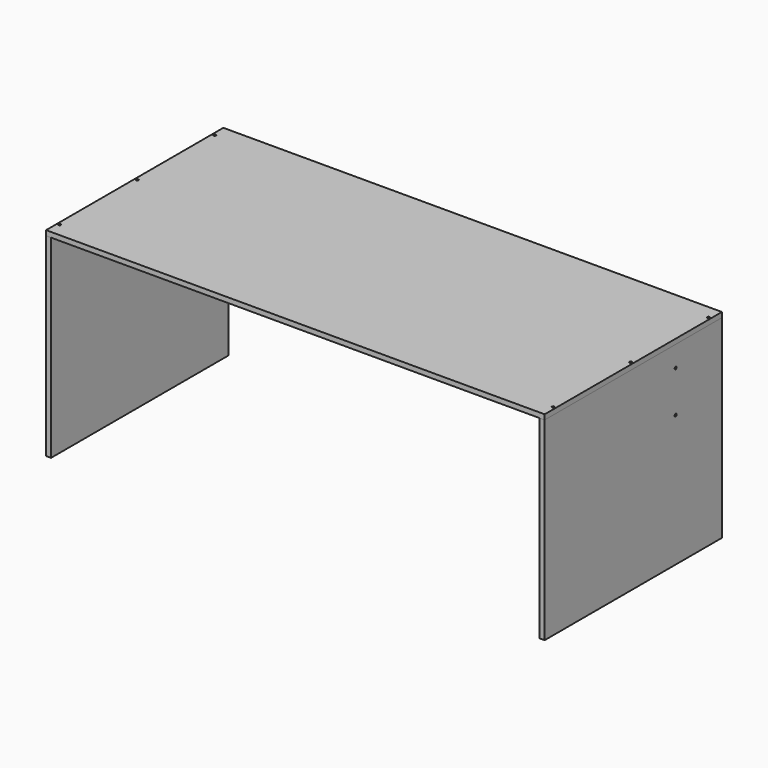
from build123d import *

# Parameters (mm, degrees)
F1_DEPTH          = 800
F0_W              = 18
F0_H              = 700
F2_DEPTH          = 800
F3_W              = 1764
F3_H              = 18
F4_DEPTH          = 300
F6_D              = 4
F6_DEPTH          = 20
F6_CSINK_D        = 8.96
F6_CSINK_ANGLE    = 90
F6_TIP            = 1.2017212381
F6_2_D            = 4
F6_2_DEPTH        = 20
F6_2_CSINK_D      = 8.96
F6_2_CSINK_ANGLE  = 90
F6_2_TIP          = 1.2017212381
F6_3_D            = 4
F6_3_DEPTH        = 20
F6_3_CSINK_D      = 8.96
F6_3_CSINK_ANGLE  = 90
F6_3_TIP          = 1.2017212381
F8_D              = 4
F8_DEPTH          = 40
F8_CSINK_D        = 8.96
F8_CSINK_ANGLE    = 90
F8_TIP            = 1.2017212381
F8_2_D            = 4
F8_2_DEPTH        = 40
F8_2_CSINK_D      = 8.96
F8_2_CSINK_ANGLE  = 90
F8_2_TIP          = 1.2017212381
F10_D             = 4
F10_DEPTH         = 40
F10_CSINK_D       = 8.96
F10_CSINK_ANGLE   = 90
F10_TIP           = 1.2017212381
F10_2_D           = 4
F10_2_DEPTH       = 40
F10_2_CSINK_D     = 8.96
F10_2_CSINK_ANGLE = 90
F10_2_TIP         = 1.2017212381
F12_D             = 3
F12_DEPTH         = 1
F12_TIP           = 0.9012909285
F12_2_D           = 3
F12_2_DEPTH       = 1
F12_2_TIP         = 0.9012909285


# Not quite as in the source:
# - a feature names something its author has since deleted; it is built from what else it names


with BuildPart() as f1:
    # F0 (on Front) → F1 (new body)
    with BuildSketch(Plane.XZ):
        Polygon((0, 18), (0, 0), (18, 0), (1782, 0), (1800, 0), (1800, 18), align=None)
    extrude(amount=-F1_DEPTH)

    # F6
    with Locations(Plane.XY.offset(18)):
        with Locations((9, 750), (9, 400), (9, 50), (1791, 750), (1791, 400), (1791, 50)):
            CounterSinkHole(F6_D / 2, F6_CSINK_D / 2, depth=F6_DEPTH, counter_sink_angle=F6_CSINK_ANGLE)
            with Locations((0, 0, -(F6_DEPTH + F6_TIP / 2))):  # 118° drill point
                Cone(0, F6_D / 2, F6_TIP, mode=Mode.SUBTRACT)


with BuildPart() as f2:
    # F0 (on Front) → F2 (new body)
    with BuildSketch(Plane.XZ):
        with Locations((9, -350)):
            Rectangle(F0_W, F0_H)
    extrude(amount=-F2_DEPTH)

    # F6#2
    with Locations(Plane.XY.offset(18)):
        with Locations((9, 750), (9, 400), (9, 50), (1791, 750), (1791, 400), (1791, 50)):
            CounterSinkHole(F6_2_D / 2, F6_2_CSINK_D / 2, depth=F6_2_DEPTH, counter_sink_angle=F6_2_CSINK_ANGLE)
            with Locations((0, 0, -(F6_2_DEPTH + F6_2_TIP / 2))):  # 118° drill point
                Cone(0, F6_2_D / 2, F6_2_TIP, mode=Mode.SUBTRACT)

    # F8
    with Locations(Plane(origin=(0, 0, 0), x_dir=(0, -1, 0), z_dir=(-1, 0, 0))):
        with Locations((-591, -75), (-591, -225)):
            CounterSinkHole(F8_D / 2, F8_CSINK_D / 2, depth=F8_DEPTH, counter_sink_angle=F8_CSINK_ANGLE)
            with Locations((0, 0, -(F8_DEPTH + F8_TIP / 2))):  # 118° drill point
                Cone(0, F8_D / 2, F8_TIP, mode=Mode.SUBTRACT)

    # F12
    with Locations(Plane(origin=(0, 0, -700), x_dir=(1, 0, 0), z_dir=(0, 0, -1))):
        with Locations((1791, -30), (1791, -770), (9, -30), (9, -770)):
            Hole(F12_D / 2, depth=F12_DEPTH)
            with Locations((0, 0, -(F12_DEPTH + F12_TIP / 2))):  # 118° drill point
                Cone(0, F12_D / 2, F12_TIP, mode=Mode.SUBTRACT)


with BuildPart() as f2b:
    # F0 (on Front) → F2, piece 2 (new body)
    with BuildSketch(Plane.XZ):
        with Locations((1791, -350)):
            Rectangle(F0_W, F0_H)
    extrude(amount=-F2_DEPTH)

    # F6#3
    with Locations(Plane.XY.offset(18)):
        with Locations((9, 750), (9, 400), (9, 50), (1791, 750), (1791, 400), (1791, 50)):
            CounterSinkHole(F6_3_D / 2, F6_3_CSINK_D / 2, depth=F6_3_DEPTH, counter_sink_angle=F6_3_CSINK_ANGLE)
            with Locations((0, 0, -(F6_3_DEPTH + F6_3_TIP / 2))):  # 118° drill point
                Cone(0, F6_3_D / 2, F6_3_TIP, mode=Mode.SUBTRACT)

    # F10
    with Locations(Plane.YZ.offset(1800)):
        with Locations((591, -75), (591, -225)):
            CounterSinkHole(F10_D / 2, F10_CSINK_D / 2, depth=F10_DEPTH, counter_sink_angle=F10_CSINK_ANGLE)
            with Locations((0, 0, -(F10_DEPTH + F10_TIP / 2))):  # 118° drill point
                Cone(0, F10_D / 2, F10_TIP, mode=Mode.SUBTRACT)

    # F12#2
    with Locations(Plane(origin=(0, 0, -700), x_dir=(1, 0, 0), z_dir=(0, 0, -1))):
        with Locations((1791, -30), (1791, -770), (9, -30), (9, -770)):
            Hole(F12_2_D / 2, depth=F12_2_DEPTH)
            with Locations((0, 0, -(F12_2_DEPTH + F12_2_TIP / 2))):  # 118° drill point
                Cone(0, F12_2_D / 2, F12_2_TIP, mode=Mode.SUBTRACT)


with BuildPart() as f4:
    # F3 (on face) → F4 (new body)
    with BuildSketch(Plane(origin=(0, 0, 0), x_dir=(1, 0, 0), z_dir=(0, 0, -1))):
        with Locations((900, -591)):
            Rectangle(F3_W, F3_H)
    extrude(amount=F4_DEPTH)

    # F8#2
    with Locations(Plane(origin=(0, 0, 0), x_dir=(0, -1, 0), z_dir=(-1, 0, 0))):
        with Locations((-591, -75), (-591, -225)):
            CounterSinkHole(F8_2_D / 2, F8_2_CSINK_D / 2, depth=F8_2_DEPTH, counter_sink_angle=F8_2_CSINK_ANGLE)
            with Locations((0, 0, -(F8_2_DEPTH + F8_2_TIP / 2))):  # 118° drill point
                Cone(0, F8_2_D / 2, F8_2_TIP, mode=Mode.SUBTRACT)

    # F10#2
    with Locations(Plane.YZ.offset(1800)):
        with Locations((591, -75), (591, -225)):
            CounterSinkHole(F10_2_D / 2, F10_2_CSINK_D / 2, depth=F10_2_DEPTH, counter_sink_angle=F10_2_CSINK_ANGLE)
            with Locations((0, 0, -(F10_2_DEPTH + F10_2_TIP / 2))):  # 118° drill point
                Cone(0, F10_2_D / 2, F10_2_TIP, mode=Mode.SUBTRACT)


solid = Compound([f1.part, f2.part, f2b.part, f4.part])
